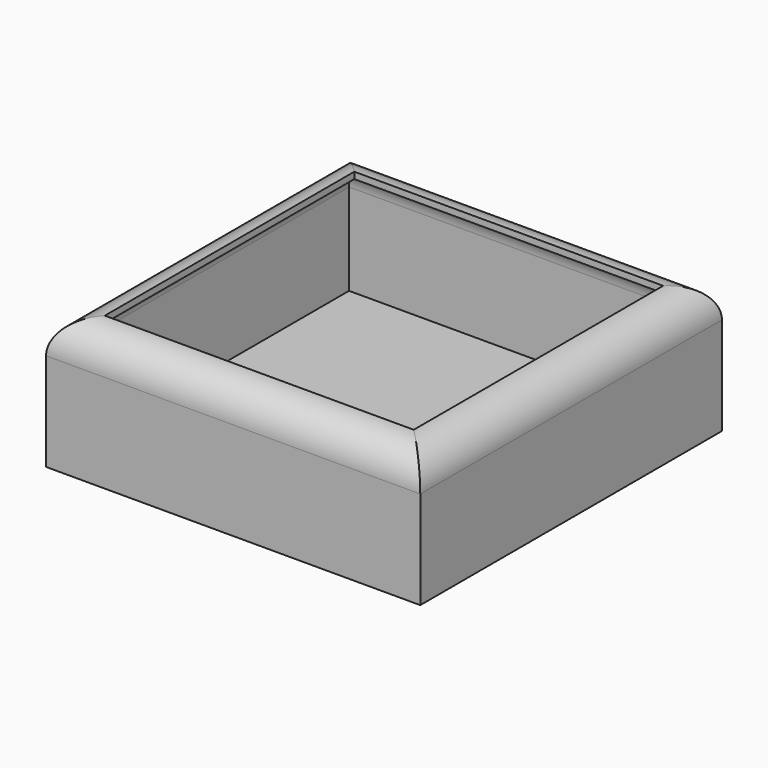
from build123d import *

# Parameters (mm, degrees)
F0_W     = 145.6201821566
F0_H     = 146.7496156693
F1_DEPTH = 50.8
F2_R     = 12.7
F3_T     = -2.54


# Not quite as in the source:
# - a shell that OpenCascade refuses in one call is made with other operations: the cavity is built on its own and cut out


with BuildPart() as f1:
    # F0 (on Top) → F1 (new body)
    with BuildSketch(Plane.XY):
        with Locations((0.0337362289, 0.0121071935)):
            Rectangle(F0_W, F0_H)
    extrude(amount=F1_DEPTH)

    # F2
    f2_edges = [f1.edges().sort_by_distance(p)[0] for p in [
        (0.033736, -73.362701, 50.8),
        (72.843827, 0.012107, 50.8),
        (0.033736, 73.386915, 50.8),
        (-72.776355, 0.012107, 50.8),
    ]]
    fillet(f2_edges, radius=F2_R)

    # F3: a shell. OpenCascade refuses it in one call, so the cavity is built on its own and cut out:
    # the body offset inwards by the wall thickness, plus a prism from it out through each open face.
    f3_core = offset(f1.part, amount=F3_T, mode=Mode.PRIVATE)
    f3_exits = [f3_core.faces().sort_by_distance(p)[0] for p in [
        (0.033736, 0.012107, 48.26),
    ]]
    add(f3_core, mode=Mode.SUBTRACT)
    extrude(f3_exits, amount=-F3_T, mode=Mode.SUBTRACT)


solid = f1.part
